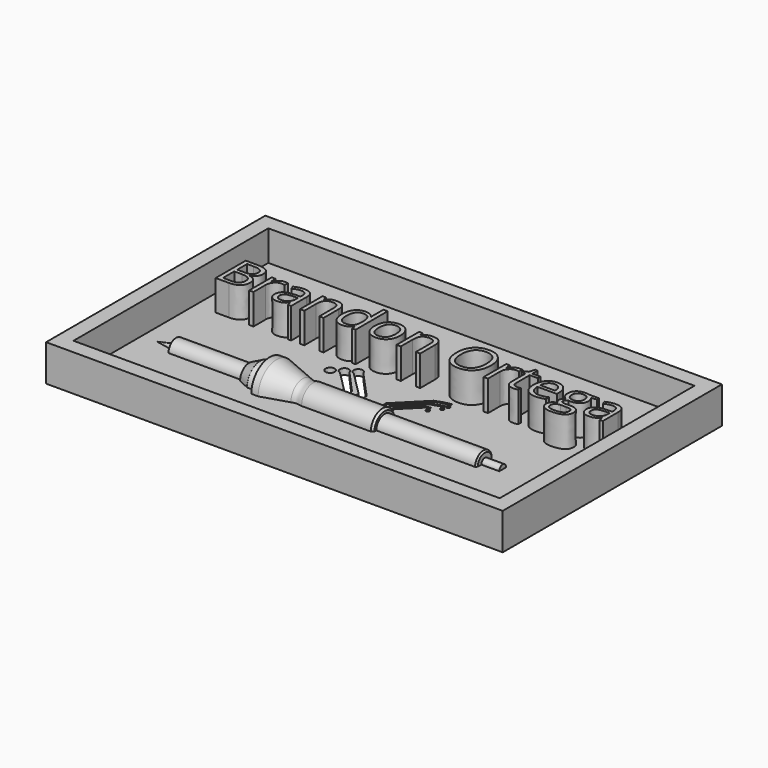
from build123d import *

# Parameters (mm, degrees)
F1_ANGLE     = 180
F0_W         = 2.8489414334
F0_H         = 1.7904182896
F2_ANGLE     = 180
F0_W_2       = 190.5
F0_H_2       = 114.3
F0_W_3       = 177.8
F0_H_3       = 101.6
F0_TEXT_SIZE = 21.9972936401
F3_DEPTH     = 2.54
F4_DEPTH     = 12.7
F5_DEPTH     = 12.7


# Not quite as in the source:
# - Text() gives the source's letters only with a copy of the font that has no kerning and outlines rounded to 1/6400 em; it was checked with that copy


with BuildPart() as f1:
    # F0 (on Top) → F1 (revolve)
    with BuildSketch(Plane.XY):
        with BuildLine():
            Line((-74.5651721954, -13.5963652283), (-82.55, -15.2098201215))
            Line((-82.55, -15.2098201215), (58.8370602846, -15.2098201215))
            Line((58.8370602846, -15.2098201215), (58.8370602846, -13.4194018319))
            Line((58.8370602846, -13.4194018319), (54.2072419855, -13.4194018319))
            Line((54.2072419855, -13.4194018319), (54.2072419855, -11.5678850561))
            Line((54.2072419855, -11.5678850561), (53.6286447975, -10.887705721))
            Line((53.6286447975, -10.887705721), (12.4287380683, -10.887705721))
            Line((12.4287380683, -10.887705721), (12.4287380683, -9.9038422616))
            Line((12.4287380683, -9.9038422616), (11.5140470523, -9.1452874751))
            Line((11.5140470523, -9.1452874751), (7.7323295531, -9.1452874751))
            Line((7.7323295531, -9.1452874751), (6.9703295531, -9.1452874751))
            Line((6.9703295531, -9.1452874751), (5.7003295531, -9.1452874751))
            Line((5.7003295531, -9.1452874751), (4.9383295531, -9.1452874751))
            Line((4.9383295531, -9.1452874751), (3.6683295531, -9.1452874751))
            Line((3.6683295531, -9.1452874751), (2.9063295531, -9.1452874751))
            Line((2.9063295531, -9.1452874751), (-5.1990439205, -9.1452874751))
            Line((-5.1990439205, -9.1452874751), (-8.3740439205, -9.1452874751))
            Line((-8.3740439205, -9.1452874751), (-10.9140439205, -9.1452874751))
            Line((-10.9140439205, -9.1452874751), (-14.0890439205, -9.1452874751))
            Line((-14.0890439205, -9.1452874751), (-16.6290439205, -9.1452874751))
            Line((-16.6290439205, -9.1452874751), (-17.3627614197, -9.1452874751))
            add(Edge.make_bspline(
                [(-21.7048861086, -9.0066427365), (-21.0124520956, -9.19988297), (-19.5884720556, -9.7925185893), (-18.2162617645, -9.1413361473), (-17.3627614197, -9.1452874751)],
                knots=[0, 0, 0, 0, 0.4911919612, 1, 1, 1, 1], degree=3))
            Line((-21.7048861086, -9.0066427365), (-32.662589103, -5.6135384366))
            Line((-32.662589103, -5.6135384366), (-35.5079583824, -5.6135384366))
            Line((-35.5079583824, -5.6135384366), (-35.5079583824, -8.2424543798))
            Line((-35.5079583824, -8.2424543798), (-39.3697954714, -8.2424543798))
            Line((-39.3697954714, -8.2424543798), (-44.1093221307, -10.5244489387))
            Line((-44.1093221307, -10.5244489387), (-44.1093221307, -11.2266018987))
            Line((-44.1093221307, -11.2266018987), (-74.5651721954, -11.2266018987))
            Line((-74.5651721954, -11.2266018987), (-74.5651721954, -13.5963652283))
        make_face()
    revolve(axis=Axis((-11.8564698577, -15.2098201215, 0), (1, 0, 0)), revolution_arc=F1_ANGLE)

    # F0 (on Top) → F2 (revolve)
    with BuildSketch(Plane.XY):
        with Locations((60.2615310013, -14.3146109767)):
            Rectangle(F0_W, F0_H)
    revolve(axis=Axis((60.2615310013, -15.2098201215, 0), (1, 0, 0)), revolution_arc=F2_ANGLE)

    # F0 (on Top) → F3 (join)
    with BuildSketch(Plane.XY):
        Rectangle(F0_W_2, F0_H_2)
        Rectangle(F0_W_3, F0_H_3, mode=Mode.SUBTRACT)
        Rectangle(F0_W_3, F0_H_3)
        with BuildLine():
            Line((-74.5651721954, -16.8232750148), (-82.55, -15.2098201215))
            Line((-82.55, -15.2098201215), (-74.5651721954, -13.5963652283))
            Line((-74.5651721954, -13.5963652283), (-74.5651721954, -11.2266018987))
            Line((-74.5651721954, -11.2266018987), (-44.1093221307, -11.2266018987))
            Line((-44.1093221307, -11.2266018987), (-44.1093221307, -10.5244489387))
            Line((-44.1093221307, -10.5244489387), (-39.3697954714, -8.2424543798))
            Line((-39.3697954714, -8.2424543798), (-35.5079583824, -8.2424543798))
            Line((-35.5079583824, -8.2424543798), (-35.5079583824, -5.6135384366))
            Line((-35.5079583824, -5.6135384366), (-32.662589103, -5.6135384366))
            Line((-32.662589103, -5.6135384366), (-21.7048861086, -9.0066427365))
            add(Edge.make_bspline(
                [(-21.7048861086, -9.0066427365), (-21.0124520956, -9.19988297), (-19.5884720556, -9.7925185893), (-18.2162617645, -9.1413361473), (-17.3627614197, -9.1452874751)],
                knots=[0, 0, 0, 0, 0.4911919612, 1, 1, 1, 1], degree=3))
            Line((-17.3627614197, -9.1452874751), (-16.6290439205, -9.1452874751))
            Line((-16.6290439205, -9.1452874751), (-14.0890439205, -9.1452874751))
            Line((-14.0890439205, -9.1452874751), (-14.0890439205, -3.3032874751))
            Line((-14.0890439205, -3.3032874751), (-22.3246965397, 4.9323651441))
            ThreePointArc((-22.3246965397, 4.9323651441), (-23.2578395891, 8.1815702533), (-20.062313494, 7.0785277481))
            Line((-20.062313494, 7.0785277481), (-10.9140439205, -3.0492874751))
            Line((-10.9140439205, -3.0492874751), (-10.9140439205, -9.1452874751))
            Line((-10.9140439205, -9.1452874751), (-8.3740439205, -9.1452874751))
            Line((-8.3740439205, -9.1452874751), (-8.3740439205, -2.7952874751))
            Line((-8.3740439205, -2.7952874751), (-18.4026051549, 7.2332737592))
            ThreePointArc((-18.4026051549, 7.2332737592), (-19.3413648826, 10.4771416844), (-16.1425614334, 9.3947344434))
            Line((-16.1425614334, 9.3947344434), (-5.1990439205, -2.5412874751))
            Line((-5.1990439205, -2.5412874751), (-5.1990439205, -9.1452874751))
            Line((-5.1990439205, -9.1452874751), (2.9063295531, -9.1452874751))
            Line((2.9063295531, -9.1452874751), (2.9063295531, -2.5412874751))
            Line((2.9063295531, -2.5412874751), (13.9043204597, 8.5183257555))
            Line((13.9043204597, 8.5183257555), (17.1510335058, 9.6937734634))
            Line((17.1510335058, 9.6937734634), (20.0589859507, 10.3021474712))
            Line((20.0589859507, 10.3021474712), (20.2566589924, 9.566233503))
            Line((20.2566589924, 9.566233503), (20.549468061, 8.7620187263))
            ThreePointArc((20.549468061, 8.7620187263), (21.0009293474, 8.5014168437), (21.1792302885, 8.0115807398))
            ThreePointArc((21.1792302885, 8.0115807398), (20.1560011796, 7.2957571913), (19.8343395992, 8.5023785029))
            Line((19.8343395992, 8.5023785029), (19.5207450243, 9.3685604613))
            Line((19.5207450243, 9.3685604613), (17.4104327689, 8.9772847877))
            Line((17.4104327689, 8.9772847877), (14.4446368983, 7.9810198702))
            Line((14.4446368983, 7.9810198702), (3.6683295531, -2.7952874751))
            Line((3.6683295531, -2.7952874751), (3.6683295531, -9.1452874751))
            Line((3.6683295531, -9.1452874751), (4.9383295531, -9.1452874751))
            Line((4.9383295531, -9.1452874751), (4.9383295531, -3.0492874751))
            Line((4.9383295531, -3.0492874751), (14.1417703069, 6.2157840132))
            Line((14.1417703069, 6.2157840132), (17.3898523031, 7.3917273391))
            Line((17.3898523031, 7.3917273391), (19.34044637, 7.947929778))
            Line((19.34044637, 7.947929778), (19.5381194117, 7.2120158098))
            Line((19.5381194117, 7.2120158098), (19.8309284803, 6.4078010331))
            ThreePointArc((19.8309284803, 6.4078010331), (20.2823897667, 6.1471991505), (20.4606907078, 5.6573630466))
            ThreePointArc((20.4606907078, 5.6573630466), (19.4374615989, 4.9415394981), (19.1158000185, 6.1481608097))
            Line((19.1158000185, 6.1481608097), (18.8022054435, 7.014342768))
            Line((18.8022054435, 7.014342768), (17.632497658, 6.6693927685))
            Line((17.632497658, 6.6693927685), (14.6805856741, 5.6769686459))
            Line((14.6805856741, 5.6769686459), (5.7003295531, -3.3032874751))
            Line((5.7003295531, -3.3032874751), (5.7003295531, -9.1452874751))
            Line((5.7003295531, -9.1452874751), (6.9703295531, -9.1452874751))
            Line((6.9703295531, -9.1452874751), (6.9703295531, -3.8112874751))
            Line((6.9703295531, -3.8112874751), (14.3754961374, 3.6554913484))
            Line((14.3754961374, 3.6554913484), (16.3270021512, 4.1796832328))
            Line((16.3270021512, 4.1796832328), (16.524675193, 3.4437692646))
            Line((16.524675193, 3.4437692646), (16.8174842615, 2.6395544879))
            ThreePointArc((16.8174842615, 2.6395544879), (17.2689455479, 2.3789526053), (17.447246489, 1.8891165014))
            ThreePointArc((17.447246489, 1.8891165014), (16.4240173801, 1.1732929529), (16.1023557997, 2.3799142645))
            Line((16.1023557997, 2.3799142645), (15.7887612248, 3.2460962229))
            Line((15.7887612248, 3.2460962229), (14.9165344499, 3.1189174217))
            Line((14.9165344499, 3.1189174217), (7.7323295531, -4.0652874751))
            Line((7.7323295531, -4.0652874751), (7.7323295531, -9.1452874751))
            Line((7.7323295531, -9.1452874751), (11.5140470523, -9.1452874751))
            Line((11.5140470523, -9.1452874751), (12.4287380683, -9.9038422616))
            Line((12.4287380683, -9.9038422616), (12.4287380683, -10.887705721))
            Line((12.4287380683, -10.887705721), (53.6286447975, -10.887705721))
            Line((53.6286447975, -10.887705721), (54.2072419855, -11.5678850561))
            Line((54.2072419855, -11.5678850561), (54.2072419855, -13.4194018319))
            Line((54.2072419855, -13.4194018319), (58.8370602846, -13.4194018319))
            Line((58.8370602846, -13.4194018319), (61.686001718, -13.4194018319))
            Line((61.686001718, -13.4194018319), (61.686001718, -15.2098201215))
            Line((61.686001718, -15.2098201215), (61.686001718, -17.0002384111))
            Line((61.686001718, -17.0002384111), (58.8370602846, -17.0002384111))
            Line((58.8370602846, -17.0002384111), (54.2072419855, -17.0002384111))
            Line((54.2072419855, -17.0002384111), (54.2072419855, -18.8517551869))
            Line((54.2072419855, -18.8517551869), (53.6286447975, -19.5319345221))
            Line((53.6286447975, -19.5319345221), (12.4287380683, -19.5319345221))
            Line((12.4287380683, -19.5319345221), (12.4287380683, -20.5157979815))
            Line((12.4287380683, -20.5157979815), (11.5140470523, -21.2743527679))
            Line((11.5140470523, -21.2743527679), (3.657140649, -21.2743527679))
            Line((3.657140649, -21.2743527679), (2.895140649, -21.2743527679))
            Line((2.895140649, -21.2743527679), (1.625140649, -21.2743527679))
            Line((1.625140649, -21.2743527679), (0.863140649, -21.2743527679))
            Line((0.863140649, -21.2743527679), (-0.406859351, -21.2743527679))
            Line((-0.406859351, -21.2743527679), (-1.168859351, -21.2743527679))
            Line((-1.168859351, -21.2743527679), (-17.3627614197, -21.2743527679))
            add(Edge.make_bspline(
                [(-21.7048861086, -21.4129975066), (-21.0124520956, -21.219757273), (-19.5884720556, -20.6271216538), (-18.2162617645, -21.2783040958), (-17.3627614197, -21.2743527679)],
                knots=[0, 0, 0, 0, 0.4911919612, 1, 1, 1, 1], degree=3))
            Line((-21.7048861086, -21.4129975066), (-32.662589103, -24.8061018065))
            Line((-32.662589103, -24.8061018065), (-35.5079583824, -24.8061018065))
            Line((-35.5079583824, -24.8061018065), (-35.5079583824, -22.1771858633))
            Line((-35.5079583824, -22.1771858633), (-39.3697954714, -22.1771858633))
            Line((-39.3697954714, -22.1771858633), (-44.1093221307, -19.8951913044))
            Line((-44.1093221307, -19.8951913044), (-44.1093221307, -19.1930383444))
            Line((-44.1093221307, -19.1930383444), (-62.366220009, -19.1930383444))
            Line((-62.366220009, -19.1930383444), (-63.128220009, -19.1930383444))
            Line((-63.128220009, -19.1930383444), (-64.398220009, -19.1930383444))
            Line((-64.398220009, -19.1930383444), (-65.160220009, -19.1930383444))
            Line((-65.160220009, -19.1930383444), (-66.430220009, -19.1930383444))
            Line((-66.430220009, -19.1930383444), (-67.192220009, -19.1930383444))
            Line((-67.192220009, -19.1930383444), (-74.5651721954, -19.1930383444))
            Line((-74.5651721954, -19.1930383444), (-74.5651721954, -16.8232750148))
        make_face(mode=Mode.SUBTRACT)
        with BuildLine():
            Line((-80.3915155616, 12.7), (-80.3915155616, 28.4040054127))
            Line((-80.3915155616, 28.4040054127), (-75.9542489851, 28.4040054127))
            add(Edge.make_bspline(
                [(-75.9542489851, 28.4040054127), (-72.8299458728, 28.4040054127), (-71.4327740189, 27.469120433)],
                knots=[0, 0, 0, 1, 1, 1], degree=2))
            add(Edge.make_bspline(
                [(-71.4327740189, 27.469120433), (-70.0356021651, 26.5342354533), (-70.0356021651, 24.5166711773)],
                knots=[0, 0, 0, 1, 1, 1], degree=2))
            add(Edge.make_bspline(
                [(-70.0356021651, 24.5166711773), (-70.0356021651, 23.1177807848), (-70.8141001353, 22.2103924222)],
                knots=[0, 0, 0, 1, 1, 1], degree=2))
            add(Edge.make_bspline(
                [(-70.8141001353, 22.2103924222), (-71.5925981055, 21.3030040595), (-73.0877266576, 21.0349120433)],
                knots=[0, 0, 0, 1, 1, 1], degree=2))
            Line((-73.0877266576, 21.0349120433), (-73.0877266576, 20.9283626522))
            add(Edge.make_bspline(
                [(-73.0877266576, 20.9283626522), (-69.509729364, 20.3165629229), (-69.509729364, 17.1682002706)],
                knots=[0, 0, 0, 1, 1, 1], degree=2))
            add(Edge.make_bspline(
                [(-69.509729364, 17.1682002706), (-69.509729364, 15.0647090663), (-70.9326792963, 13.8823545332)],
                knots=[0, 0, 0, 1, 1, 1], degree=2))
            add(Edge.make_bspline(
                [(-70.9326792963, 13.8823545332), (-72.3556292287, 12.7), (-74.9128146143, 12.7)],
                knots=[0, 0, 0, 1, 1, 1], degree=2))
            Line((-74.9128146143, 12.7), (-80.3915155616, 12.7))
        make_face(mode=Mode.SUBTRACT)
        with BuildLine():
            add(Edge.make_bspline(
                [(-63.0652097429, 24.0646955345), (-62.1406359946, 24.6885250338), (-61.0338971583, 24.6885250338)],
                knots=[0, 0, 0, 1, 1, 1], degree=2))
            add(Edge.make_bspline(
                [(-61.0338971583, 24.6885250338), (-60.2502435724, 24.6885250338), (-59.6281326116, 24.5579161028)],
                knots=[0, 0, 0, 1, 1, 1], degree=2))
            Line((-59.6281326116, 24.5579161028), (-59.8756021651, 22.9046820027))
            add(Edge.make_bspline(
                [(-59.8756021651, 22.9046820027), (-60.6042625169, 23.0662246279), (-61.1645060893, 23.0662246279)],
                knots=[0, 0, 0, 1, 1, 1], degree=2))
            add(Edge.make_bspline(
                [(-61.1645060893, 23.0662246279), (-62.5943301759, 23.0662246279), (-63.6082679296, 21.9062110961)],
                knots=[0, 0, 0, 1, 1, 1], degree=2))
            add(Edge.make_bspline(
                [(-63.6082679296, 21.9062110961), (-64.6222056834, 20.7461975643), (-64.6222056834, 19.0173477673)],
                knots=[0, 0, 0, 1, 1, 1], degree=2))
            Line((-64.6222056834, 19.0173477673), (-64.6222056834, 12.7))
            Line((-64.6222056834, 12.7), (-66.4060487145, 12.7))
            Line((-66.4060487145, 12.7), (-66.4060487145, 24.4719891746))
            Line((-66.4060487145, 24.4719891746), (-64.9349797023, 24.4719891746))
            Line((-64.9349797023, 24.4719891746), (-64.7287550744, 22.2928822733))
            Line((-64.7287550744, 22.2928822733), (-64.6428281461, 22.2928822733))
            add(Edge.make_bspline(
                [(-64.6428281461, 22.2928822733), (-63.9897834912, 23.4408660352), (-63.0652097429, 24.0646955345)],
                knots=[0, 0, 0, 1, 1, 1], degree=2))
        make_face(mode=Mode.SUBTRACT)
        with BuildLine():
            Line((-48.8632070365, 12.7), (-50.1864817321, 12.7))
            Line((-50.1864817321, 12.7), (-50.5405006766, 14.3772936401))
            Line((-50.5405006766, 14.3772936401), (-50.6264276049, 14.3772936401))
            add(Edge.make_bspline(
                [(-50.6264276049, 14.3772936401), (-51.5063193505, 13.2705548038), (-52.3810554804, 12.8770094723)],
                knots=[0, 0, 0, 1, 1, 1], degree=2))
            add(Edge.make_bspline(
                [(-52.3810554804, 12.8770094723), (-53.2557916103, 12.4834641407), (-54.5687550744, 12.4834641407)],
                knots=[0, 0, 0, 1, 1, 1], degree=2))
            add(Edge.make_bspline(
                [(-54.5687550744, 12.4834641407), (-56.3182273342, 12.4834641407), (-57.3115426252, 13.3874154263)],
                knots=[0, 0, 0, 1, 1, 1], degree=2))
            add(Edge.make_bspline(
                [(-57.3115426252, 13.3874154263), (-58.3048579161, 14.2913667118), (-58.3048579161, 15.9549120433)],
                knots=[0, 0, 0, 1, 1, 1], degree=2))
            add(Edge.make_bspline(
                [(-58.3048579161, 15.9549120433), (-58.3048579161, 19.5191610284), (-52.6027469553, 19.691014885)],
                knots=[0, 0, 0, 1, 1, 1], degree=2))
            Line((-52.6027469553, 19.691014885), (-50.6058051421, 19.7563193505))
            Line((-50.6058051421, 19.7563193505), (-50.6058051421, 20.4884167794))
            add(Edge.make_bspline(
                [(-50.6058051421, 20.4884167794), (-50.6058051421, 21.8735588633), (-51.2004194858, 22.5334776725)],
                knots=[0, 0, 0, 1, 1, 1], degree=2))
            add(Edge.make_bspline(
                [(-51.2004194858, 22.5334776725), (-51.7950338295, 23.1933964817), (-53.1079972936, 23.1933964817)],
                knots=[0, 0, 0, 1, 1, 1], degree=2))
            add(Edge.make_bspline(
                [(-53.1079972936, 23.1933964817), (-54.5790663058, 23.1933964817), (-56.4350879567, 22.2928822733)],
                knots=[0, 0, 0, 1, 1, 1], degree=2))
            Line((-56.4350879567, 22.2928822733), (-56.9850202977, 23.6574018945))
            add(Edge.make_bspline(
                [(-56.9850202977, 23.6574018945), (-56.1154397835, 24.1282814614), (-55.0791610284, 24.3963734777)],
                knots=[0, 0, 0, 1, 1, 1], degree=2))
            add(Edge.make_bspline(
                [(-55.0791610284, 24.3963734777), (-54.0428822733, 24.6644654939), (-52.9980108254, 24.6644654939)],
                knots=[0, 0, 0, 1, 1, 1], degree=2))
            add(Edge.make_bspline(
                [(-52.9980108254, 24.6644654939), (-50.8945196211, 24.6644654939), (-49.8788633288, 23.7312990528)],
                knots=[0, 0, 0, 1, 1, 1], degree=2))
            add(Edge.make_bspline(
                [(-49.8788633288, 23.7312990528), (-48.8632070365, 22.7981326116), (-48.8632070365, 20.7358863329)],
                knots=[0, 0, 0, 1, 1, 1], degree=2))
            Line((-48.8632070365, 20.7358863329), (-48.8632070365, 12.7))
        make_face(mode=Mode.SUBTRACT)
        with BuildLine():
            ThreePointArc((-26.2389803515, 2.3696489559), (-27.1644583182, 5.626112764), (-23.9736375963, 4.4948616332))
            ThreePointArc((-23.9736375963, 4.4948616332), (-23.960471465, 4.3661239156), (-23.9560759934, 4.236789362))
            ThreePointArc((-23.9560759934, 4.236789362), (-24.6550251657, 2.7621821597), (-26.2389803515, 2.3696489559))
        make_face(mode=Mode.SUBTRACT)
        with BuildLine():
            Line((-35.3520568336, 12.7), (-37.1358998647, 12.7))
            Line((-37.1358998647, 12.7), (-37.1358998647, 20.3165629229))
            add(Edge.make_bspline(
                [(-37.1358998647, 20.3165629229), (-37.1358998647, 21.7532611637), (-37.7906630582, 22.4630175913)],
                knots=[0, 0, 0, 1, 1, 1], degree=2))
            add(Edge.make_bspline(
                [(-37.7906630582, 22.4630175913), (-38.4454262517, 23.1727740189), (-39.8443166441, 23.1727740189)],
                knots=[0, 0, 0, 1, 1, 1], degree=2))
            add(Edge.make_bspline(
                [(-39.8443166441, 23.1727740189), (-41.6900270636, 23.1727740189), (-42.5492963464, 22.1743031123)],
                knots=[0, 0, 0, 1, 1, 1], degree=2))
            add(Edge.make_bspline(
                [(-42.5492963464, 22.1743031123), (-43.4085656292, 21.1758322057), (-43.4085656292, 18.8764276049)],
                knots=[0, 0, 0, 1, 1, 1], degree=2))
            Line((-43.4085656292, 18.8764276049), (-43.4085656292, 12.7))
            Line((-43.4085656292, 12.7), (-45.1924086604, 12.7))
            Line((-45.1924086604, 12.7), (-45.1924086604, 24.4719891746))
            Line((-45.1924086604, 24.4719891746), (-43.741962111, 24.4719891746))
            Line((-43.741962111, 24.4719891746), (-43.4532476319, 22.86))
            Line((-43.4532476319, 22.86), (-43.3673207037, 22.86))
            add(Edge.make_bspline(
                [(-43.3673207037, 22.86), (-42.8173883627, 23.7295805142), (-41.8292286874, 24.209052774)],
                knots=[0, 0, 0, 1, 1, 1], degree=2))
            add(Edge.make_bspline(
                [(-41.8292286874, 24.209052774), (-40.8410690122, 24.6885250338), (-39.6277807848, 24.6885250338)],
                knots=[0, 0, 0, 1, 1, 1], degree=2))
            add(Edge.make_bspline(
                [(-39.6277807848, 24.6885250338), (-37.5002300406, 24.6885250338), (-36.4261434371, 23.6625575101)],
                knots=[0, 0, 0, 1, 1, 1], degree=2))
            add(Edge.make_bspline(
                [(-36.4261434371, 23.6625575101), (-35.3520568336, 22.6365899865), (-35.3520568336, 20.3784303112)],
                knots=[0, 0, 0, 1, 1, 1], degree=2))
            Line((-35.3520568336, 20.3784303112), (-35.3520568336, 12.7))
        make_face(mode=Mode.SUBTRACT)
        with BuildLine():
            Line((-23.4425845737, 12.7), (-23.6797428958, 14.2776184032))
            Line((-23.6797428958, 14.2776184032), (-23.7759810555, 14.2776184032))
            add(Edge.make_bspline(
                [(-23.7759810555, 14.2776184032), (-25.0098917456, 12.4834641407), (-27.4708389716, 12.4834641407)],
                knots=[0, 0, 0, 1, 1, 1], degree=2))
            add(Edge.make_bspline(
                [(-27.4708389716, 12.4834641407), (-29.7805548038, 12.4834641407), (-31.0643031123, 14.0628010825)],
                knots=[0, 0, 0, 1, 1, 1], degree=2))
            add(Edge.make_bspline(
                [(-31.0643031123, 14.0628010825), (-32.3480514208, 15.6421380244), (-32.3480514208, 18.5533423545)],
                knots=[0, 0, 0, 1, 1, 1], degree=2))
            add(Edge.make_bspline(
                [(-32.3480514208, 18.5533423545), (-32.3480514208, 21.4645466847), (-31.0591474966, 23.0765358593)],
                knots=[0, 0, 0, 1, 1, 1], degree=2))
            add(Edge.make_bspline(
                [(-31.0591474966, 23.0765358593), (-29.7702435724, 24.6885250338), (-27.4708389716, 24.6885250338)],
                knots=[0, 0, 0, 1, 1, 1], degree=2))
            add(Edge.make_bspline(
                [(-27.4708389716, 24.6885250338), (-25.0751962111, 24.6885250338), (-23.7966035183, 22.9459269283)],
                knots=[0, 0, 0, 1, 1, 1], degree=2))
            Line((-23.7966035183, 22.9459269283), (-23.6556833559, 22.9459269283))
            Line((-23.6556833559, 22.9459269283), (-23.7312990528, 23.7948849797))
            Line((-23.7312990528, 23.7948849797), (-23.7759810555, 24.6232205683))
            Line((-23.7759810555, 24.6232205683), (-23.7759810555, 29.4145060893))
            Line((-23.7759810555, 29.4145060893), (-21.9921380244, 29.4145060893))
            Line((-21.9921380244, 29.4145060893), (-21.9921380244, 12.7))
            Line((-21.9921380244, 12.7), (-23.4425845737, 12.7))
        make_face(mode=Mode.SUBTRACT)
        with BuildLine():
            add(Edge.make_bspline(
                [(-9.5069553451, 23.0438836265), (-8.05135318, 21.3992422192), (-8.05135318, 18.5980243572)],
                knots=[0, 0, 0, 1, 1, 1], degree=2))
            add(Edge.make_bspline(
                [(-8.05135318, 18.5980243572), (-8.05135318, 15.7177537212), (-9.5000811908, 14.100608931)],
                knots=[0, 0, 0, 1, 1, 1], degree=2))
            add(Edge.make_bspline(
                [(-9.5000811908, 14.100608931), (-10.9488092016, 12.4834641407), (-13.5059945873, 12.4834641407)],
                knots=[0, 0, 0, 1, 1, 1], degree=2))
            add(Edge.make_bspline(
                [(-13.5059945873, 12.4834641407), (-15.0870500677, 12.4834641407), (-16.3106495264, 13.2258728011)],
                knots=[0, 0, 0, 1, 1, 1], degree=2))
            add(Edge.make_bspline(
                [(-16.3106495264, 13.2258728011), (-17.5342489851, 13.9682814614), (-18.2010419486, 15.3534235453)],
                knots=[0, 0, 0, 1, 1, 1], degree=2))
            add(Edge.make_bspline(
                [(-18.2010419486, 15.3534235453), (-18.867834912, 16.7385656292), (-18.867834912, 18.5980243572)],
                knots=[0, 0, 0, 1, 1, 1], degree=2))
            add(Edge.make_bspline(
                [(-18.867834912, 18.5980243572), (-18.867834912, 21.4748579161), (-17.427699594, 23.081691475)],
                knots=[0, 0, 0, 1, 1, 1], degree=2))
            add(Edge.make_bspline(
                [(-17.427699594, 23.081691475), (-15.987564276, 24.6885250338), (-13.4303788904, 24.6885250338)],
                knots=[0, 0, 0, 1, 1, 1], degree=2))
            add(Edge.make_bspline(
                [(-13.4303788904, 24.6885250338), (-10.9625575101, 24.6885250338), (-9.5069553451, 23.0438836265)],
                knots=[0, 0, 0, 1, 1, 1], degree=2))
        make_face(mode=Mode.SUBTRACT)
        with BuildLine():
            Line((4.9167388363, 12.7), (3.1328958051, 12.7))
            Line((3.1328958051, 12.7), (3.1328958051, 20.3165629229))
            add(Edge.make_bspline(
                [(3.1328958051, 20.3165629229), (3.1328958051, 21.7532611637), (2.4781326116, 22.4630175913)],
                knots=[0, 0, 0, 1, 1, 1], degree=2))
            add(Edge.make_bspline(
                [(2.4781326116, 22.4630175913), (1.8233694181, 23.1727740189), (0.4244790257, 23.1727740189)],
                knots=[0, 0, 0, 1, 1, 1], degree=2))
            add(Edge.make_bspline(
                [(0.4244790257, 23.1727740189), (-1.4212313938, 23.1727740189), (-2.2805006766, 22.1743031123)],
                knots=[0, 0, 0, 1, 1, 1], degree=2))
            add(Edge.make_bspline(
                [(-2.2805006766, 22.1743031123), (-3.1397699594, 21.1758322057), (-3.1397699594, 18.8764276049)],
                knots=[0, 0, 0, 1, 1, 1], degree=2))
            Line((-3.1397699594, 18.8764276049), (-3.1397699594, 12.7))
            Line((-3.1397699594, 12.7), (-4.9236129905, 12.7))
            Line((-4.9236129905, 12.7), (-4.9236129905, 24.4719891746))
            Line((-4.9236129905, 24.4719891746), (-3.4731664411, 24.4719891746))
            Line((-3.4731664411, 24.4719891746), (-3.1844519621, 22.86))
            Line((-3.1844519621, 22.86), (-3.0985250338, 22.86))
            add(Edge.make_bspline(
                [(-3.0985250338, 22.86), (-2.5485926928, 23.7295805142), (-1.5604330176, 24.209052774)],
                knots=[0, 0, 0, 1, 1, 1], degree=2))
            add(Edge.make_bspline(
                [(-1.5604330176, 24.209052774), (-0.5722733424, 24.6885250338), (0.641014885, 24.6885250338)],
                knots=[0, 0, 0, 1, 1, 1], degree=2))
            add(Edge.make_bspline(
                [(0.641014885, 24.6885250338), (2.7685656292, 24.6885250338), (3.8426522327, 23.6625575101)],
                knots=[0, 0, 0, 1, 1, 1], degree=2))
            add(Edge.make_bspline(
                [(3.8426522327, 23.6625575101), (4.9167388363, 22.6365899865), (4.9167388363, 20.3784303112)],
                knots=[0, 0, 0, 1, 1, 1], degree=2))
            Line((4.9167388363, 20.3784303112), (4.9167388363, 12.7))
        make_face(mode=Mode.SUBTRACT)
        with BuildLine():
            add(Edge.make_bspline(
                [(26.2919215156, 26.5033017591), (28.1926251691, 24.3551285521), (28.1926251691, 20.5743437077)],
                knots=[0, 0, 0, 1, 1, 1], degree=2))
            add(Edge.make_bspline(
                [(28.1926251691, 20.5743437077), (28.1926251691, 16.8038700947), (26.2850473613, 14.6436671177)],
                knots=[0, 0, 0, 1, 1, 1], degree=2))
            add(Edge.make_bspline(
                [(26.2850473613, 14.6436671177), (24.3774695535, 12.4834641407), (20.9850744249, 12.4834641407)],
                knots=[0, 0, 0, 1, 1, 1], degree=2))
            add(Edge.make_bspline(
                [(20.9850744249, 12.4834641407), (17.5170635995, 12.4834641407), (15.631826793, 14.6058592693)],
                knots=[0, 0, 0, 1, 1, 1], degree=2))
            add(Edge.make_bspline(
                [(15.631826793, 14.6058592693), (13.7465899865, 16.7282543978), (13.7465899865, 20.5949661705)],
                knots=[0, 0, 0, 1, 1, 1], degree=2))
            add(Edge.make_bspline(
                [(13.7465899865, 20.5949661705), (13.7465899865, 24.430744249), (15.6369824087, 26.5411096076)],
                knots=[0, 0, 0, 1, 1, 1], degree=2))
            add(Edge.make_bspline(
                [(15.6369824087, 26.5411096076), (17.5273748309, 28.6514749662), (21.0056968877, 28.6514749662)],
                knots=[0, 0, 0, 1, 1, 1], degree=2))
            add(Edge.make_bspline(
                [(21.0056968877, 28.6514749662), (24.391217862, 28.6514749662), (26.2919215156, 26.5033017591)],
                knots=[0, 0, 0, 1, 1, 1], degree=2))
        make_face(mode=Mode.SUBTRACT)
        with BuildLine():
            add(Edge.make_bspline(
                [(34.7643166441, 24.0646955345), (35.6888903924, 24.6885250338), (36.7956292287, 24.6885250338)],
                knots=[0, 0, 0, 1, 1, 1], degree=2))
            add(Edge.make_bspline(
                [(36.7956292287, 24.6885250338), (37.5792828146, 24.6885250338), (38.2013937754, 24.5579161028)],
                knots=[0, 0, 0, 1, 1, 1], degree=2))
            Line((38.2013937754, 24.5579161028), (37.9539242219, 22.9046820027))
            add(Edge.make_bspline(
                [(37.9539242219, 22.9046820027), (37.2252638701, 23.0662246279), (36.6650202977, 23.0662246279)],
                knots=[0, 0, 0, 1, 1, 1], degree=2))
            add(Edge.make_bspline(
                [(36.6650202977, 23.0662246279), (35.2351962111, 23.0662246279), (34.2212584574, 21.9062110961)],
                knots=[0, 0, 0, 1, 1, 1], degree=2))
            add(Edge.make_bspline(
                [(34.2212584574, 21.9062110961), (33.2073207037, 20.7461975643), (33.2073207037, 19.0173477673)],
                knots=[0, 0, 0, 1, 1, 1], degree=2))
            Line((33.2073207037, 19.0173477673), (33.2073207037, 12.7))
            Line((33.2073207037, 12.7), (31.4234776725, 12.7))
            Line((31.4234776725, 12.7), (31.4234776725, 24.4719891746))
            Line((31.4234776725, 24.4719891746), (32.8945466847, 24.4719891746))
            Line((32.8945466847, 24.4719891746), (33.1007713126, 22.2928822733))
            Line((33.1007713126, 22.2928822733), (33.1866982409, 22.2928822733))
            add(Edge.make_bspline(
                [(33.1866982409, 22.2928822733), (33.8397428958, 23.4408660352), (34.7643166441, 24.0646955345)],
                knots=[0, 0, 0, 1, 1, 1], degree=2))
        make_face(mode=Mode.SUBTRACT)
        with BuildLine():
            add(Edge.make_bspline(
                [(42.8208254398, 14.5268064953), (43.3260757781, 13.95797023), (44.2059675237, 13.95797023)],
                knots=[0, 0, 0, 1, 1, 1], degree=2))
            add(Edge.make_bspline(
                [(44.2059675237, 13.95797023), (44.6802841678, 13.95797023), (45.1202300406, 14.0267117727)],
                knots=[0, 0, 0, 1, 1, 1], degree=2))
            add(Edge.make_bspline(
                [(45.1202300406, 14.0267117727), (45.5601759134, 14.0954533153), (45.8179566982, 14.1710690122)],
                knots=[0, 0, 0, 1, 1, 1], degree=2))
            Line((45.8179566982, 14.1710690122), (45.8179566982, 12.8065493911))
            add(Edge.make_bspline(
                [(45.8179566982, 12.8065493911), (45.5292422192, 12.6690663058), (44.9655615697, 12.5762652233)],
                knots=[0, 0, 0, 1, 1, 1], degree=2))
            add(Edge.make_bspline(
                [(44.9655615697, 12.5762652233), (44.4018809202, 12.4834641407), (43.9481867388, 12.4834641407)],
                knots=[0, 0, 0, 1, 1, 1], degree=2))
            add(Edge.make_bspline(
                [(43.9481867388, 12.4834641407), (40.5351691475, 12.4834641407), (40.5351691475, 16.0820838972)],
                knots=[0, 0, 0, 1, 1, 1], degree=2))
            Line((40.5351691475, 16.0820838972), (40.5351691475, 23.0868470907))
            Line((40.5351691475, 23.0868470907), (38.847564276, 23.0868470907))
            Line((38.847564276, 23.0868470907), (38.847564276, 23.9461163735))
            Line((38.847564276, 23.9461163735), (40.5351691475, 24.6885250338))
            Line((40.5351691475, 24.6885250338), (41.2844519621, 27.2010284168))
            Line((41.2844519621, 27.2010284168), (42.3155751015, 27.2010284168))
            Line((42.3155751015, 27.2010284168), (42.3155751015, 24.4719891746))
            Line((42.3155751015, 24.4719891746), (45.73202977, 24.4719891746))
            Line((45.73202977, 24.4719891746), (45.73202977, 23.0868470907))
            Line((45.73202977, 23.0868470907), (42.3155751015, 23.0868470907))
            Line((42.3155751015, 23.0868470907), (42.3155751015, 16.157699594))
            add(Edge.make_bspline(
                [(42.3155751015, 16.157699594), (42.3155751015, 15.0956427605), (42.8208254398, 14.5268064953)],
                knots=[0, 0, 0, 1, 1, 1], degree=2))
        make_face(mode=Mode.SUBTRACT)
        with BuildLine():
            add(Edge.make_bspline(
                [(55.1771177267, 12.6621921516), (54.3350338295, 12.4834641407), (53.142368065, 12.4834641407)],
                knots=[0, 0, 0, 1, 1, 1], degree=2))
            add(Edge.make_bspline(
                [(53.142368065, 12.4834641407), (50.5336265223, 12.4834641407), (49.0230311231, 14.0748308525)],
                knots=[0, 0, 0, 1, 1, 1], degree=2))
            add(Edge.make_bspline(
                [(49.0230311231, 14.0748308525), (47.512435724, 15.6661975643), (47.512435724, 18.488037889)],
                knots=[0, 0, 0, 1, 1, 1], degree=2))
            add(Edge.make_bspline(
                [(47.512435724, 18.488037889), (47.512435724, 21.3373748309), (48.9147631935, 23.0129499323)],
                knots=[0, 0, 0, 1, 1, 1], degree=2))
            add(Edge.make_bspline(
                [(48.9147631935, 23.0129499323), (50.3170906631, 24.6885250338), (52.6817997294, 24.6885250338)],
                knots=[0, 0, 0, 1, 1, 1], degree=2))
            add(Edge.make_bspline(
                [(52.6817997294, 24.6885250338), (54.8918403248, 24.6885250338), (56.180744249, 23.2329228687)],
                knots=[0, 0, 0, 1, 1, 1], degree=2))
            add(Edge.make_bspline(
                [(56.180744249, 23.2329228687), (57.4696481732, 21.7773207037), (57.4696481732, 19.3919891746)],
                knots=[0, 0, 0, 1, 1, 1], degree=2))
            Line((57.4696481732, 19.3919891746), (57.4696481732, 18.2646278755))
            Line((57.4696481732, 18.2646278755), (49.3615832206, 18.2646278755))
            add(Edge.make_bspline(
                [(49.3615832206, 18.2646278755), (49.4165764547, 16.1920703654), (50.4098917456, 15.1179837618)],
                knots=[0, 0, 0, 1, 1, 1], degree=2))
            add(Edge.make_bspline(
                [(50.4098917456, 15.1179837618), (51.4032070365, 14.0438971583), (53.2076725304, 14.0438971583)],
                knots=[0, 0, 0, 1, 1, 1], degree=2))
            add(Edge.make_bspline(
                [(53.2076725304, 14.0438971583), (55.108376184, 14.0438971583), (56.9643978349, 14.8378619756)],
                knots=[0, 0, 0, 1, 1, 1], degree=2))
            Line((56.9643978349, 14.8378619756), (56.9643978349, 13.2464952639))
            add(Edge.make_bspline(
                [(56.9643978349, 13.2464952639), (56.0192016238, 12.8409201624), (55.1771177267, 12.6621921516)],
                knots=[0, 0, 0, 1, 1, 1], degree=2))
        make_face(mode=Mode.SUBTRACT)
        with BuildLine():
            Line((66.0760893099, 24.4719891746), (70.1455886333, 24.4719891746))
            Line((70.1455886333, 24.4719891746), (70.1455886333, 23.3446278755))
            Line((70.1455886333, 23.3446278755), (67.9664817321, 23.0868470907))
            add(Edge.make_bspline(
                [(67.9664817321, 23.0868470907), (68.2655074425, 22.7122056834), (68.5026657645, 22.1038430311)],
                knots=[0, 0, 0, 1, 1, 1], degree=2))
            add(Edge.make_bspline(
                [(68.5026657645, 22.1038430311), (68.7398240866, 21.4954803789), (68.7398240866, 20.7358863329)],
                knots=[0, 0, 0, 1, 1, 1], degree=2))
            add(Edge.make_bspline(
                [(68.7398240866, 20.7358863329), (68.7398240866, 19.0035994587), (67.5574695535, 17.9724763194)],
                knots=[0, 0, 0, 1, 1, 1], degree=2))
            add(Edge.make_bspline(
                [(67.5574695535, 17.9724763194), (66.3751150203, 16.94135318), (64.3128687415, 16.94135318)],
                knots=[0, 0, 0, 1, 1, 1], degree=2))
            add(Edge.make_bspline(
                [(64.3128687415, 16.94135318), (63.7869959405, 16.94135318), (63.3264276049, 17.0272801083)],
                knots=[0, 0, 0, 1, 1, 1], degree=2))
            add(Edge.make_bspline(
                [(63.3264276049, 17.0272801083), (62.1887550744, 16.4257916103), (62.1887550744, 15.5149661705)],
                knots=[0, 0, 0, 1, 1, 1], degree=2))
            add(Edge.make_bspline(
                [(62.1887550744, 15.5149661705), (62.1887550744, 15.030338295), (62.5857374831, 14.8000541272)],
                knots=[0, 0, 0, 1, 1, 1], degree=2))
            add(Edge.make_bspline(
                [(62.5857374831, 14.8000541272), (62.9827198917, 14.5697699594), (63.9485385656, 14.5697699594)],
                knots=[0, 0, 0, 1, 1, 1], degree=2))
            Line((63.9485385656, 14.5697699594), (66.0314073072, 14.5697699594))
            add(Edge.make_bspline(
                [(66.0314073072, 14.5697699594), (67.9458592693, 14.5697699594), (68.9701082544, 13.7637753721)],
                knots=[0, 0, 0, 1, 1, 1], degree=2))
            add(Edge.make_bspline(
                [(68.9701082544, 13.7637753721), (69.9943572395, 12.9577807848), (69.9943572395, 11.4214073072)],
                knots=[0, 0, 0, 1, 1, 1], degree=2))
            add(Edge.make_bspline(
                [(69.9943572395, 11.4214073072), (69.9943572395, 9.4657104195), (68.4270500677, 8.4397428958)],
                knots=[0, 0, 0, 1, 1, 1], degree=2))
            add(Edge.make_bspline(
                [(68.4270500677, 8.4397428958), (66.8597428958, 7.4137753721), (63.852300406, 7.4137753721)],
                knots=[0, 0, 0, 1, 1, 1], degree=2))
            add(Edge.make_bspline(
                [(63.852300406, 7.4137753721), (61.5425845737, 7.4137753721), (60.291488498, 8.2730446549)],
                knots=[0, 0, 0, 1, 1, 1], degree=2))
            add(Edge.make_bspline(
                [(60.291488498, 8.2730446549), (59.0403924222, 9.1323139378), (59.0403924222, 10.7030581867)],
                knots=[0, 0, 0, 1, 1, 1], degree=2))
            add(Edge.make_bspline(
                [(59.0403924222, 10.7030581867), (59.0403924222, 11.7754262517), (59.7278078484, 12.5607983762)],
                knots=[0, 0, 0, 1, 1, 1], degree=2))
            add(Edge.make_bspline(
                [(59.7278078484, 12.5607983762), (60.4152232747, 13.3461705007), (61.6594451962, 13.6245737483)],
                knots=[0, 0, 0, 1, 1, 1], degree=2))
            add(Edge.make_bspline(
                [(61.6594451962, 13.6245737483), (61.209188092, 13.8273612991), (60.9032882273, 14.2569959405)],
                knots=[0, 0, 0, 1, 1, 1], degree=2))
            add(Edge.make_bspline(
                [(60.9032882273, 14.2569959405), (60.5973883627, 14.6866305819), (60.5973883627, 15.2571853857)],
                knots=[0, 0, 0, 1, 1, 1], degree=2))
            add(Edge.make_bspline(
                [(60.5973883627, 15.2571853857), (60.5973883627, 15.8999188092), (60.9410960758, 16.3845466847)],
                knots=[0, 0, 0, 1, 1, 1], degree=2))
            add(Edge.make_bspline(
                [(60.9410960758, 16.3845466847), (61.2848037889, 16.8691745602), (62.0272124493, 17.3194316644)],
                knots=[0, 0, 0, 1, 1, 1], degree=2))
            add(Edge.make_bspline(
                [(62.0272124493, 17.3194316644), (61.1129499323, 17.6940730717), (60.5389580514, 18.5963058187)],
                knots=[0, 0, 0, 1, 1, 1], degree=2))
            add(Edge.make_bspline(
                [(60.5389580514, 18.5963058187), (59.9649661705, 19.4985385656), (59.9649661705, 20.660270636)],
                knots=[0, 0, 0, 1, 1, 1], degree=2))
            add(Edge.make_bspline(
                [(59.9649661705, 20.660270636), (59.9649661705, 22.5919079838), (61.1249797023, 23.6402165088)],
                knots=[0, 0, 0, 1, 1, 1], degree=2))
            add(Edge.make_bspline(
                [(61.1249797023, 23.6402165088), (62.2849932341, 24.6885250338), (64.4091069012, 24.6885250338)],
                knots=[0, 0, 0, 1, 1, 1], degree=2))
            add(Edge.make_bspline(
                [(64.4091069012, 24.6885250338), (65.3336806495, 24.6885250338), (66.0760893099, 24.4719891746)],
                knots=[0, 0, 0, 1, 1, 1], degree=2))
        make_face(mode=Mode.SUBTRACT)
        with BuildLine():
            Line((81.1236129905, 12.7), (79.800338295, 12.7))
            Line((79.800338295, 12.7), (79.4463193505, 14.3772936401))
            Line((79.4463193505, 14.3772936401), (79.3603924222, 14.3772936401))
            add(Edge.make_bspline(
                [(79.3603924222, 14.3772936401), (78.4805006766, 13.2705548038), (77.6057645467, 12.8770094723)],
                knots=[0, 0, 0, 1, 1, 1], degree=2))
            add(Edge.make_bspline(
                [(77.6057645467, 12.8770094723), (76.7310284168, 12.4834641407), (75.4180649526, 12.4834641407)],
                knots=[0, 0, 0, 1, 1, 1], degree=2))
            add(Edge.make_bspline(
                [(75.4180649526, 12.4834641407), (73.6685926928, 12.4834641407), (72.6752774019, 13.3874154263)],
                knots=[0, 0, 0, 1, 1, 1], degree=2))
            add(Edge.make_bspline(
                [(72.6752774019, 13.3874154263), (71.681962111, 14.2913667118), (71.681962111, 15.9549120433)],
                knots=[0, 0, 0, 1, 1, 1], degree=2))
            add(Edge.make_bspline(
                [(71.681962111, 15.9549120433), (71.681962111, 19.5191610284), (77.3840730717, 19.691014885)],
                knots=[0, 0, 0, 1, 1, 1], degree=2))
            Line((77.3840730717, 19.691014885), (79.381014885, 19.7563193505))
            Line((79.381014885, 19.7563193505), (79.381014885, 20.4884167794))
            add(Edge.make_bspline(
                [(79.381014885, 20.4884167794), (79.381014885, 21.8735588633), (78.7864005413, 22.5334776725)],
                knots=[0, 0, 0, 1, 1, 1], degree=2))
            add(Edge.make_bspline(
                [(78.7864005413, 22.5334776725), (78.1917861976, 23.1933964817), (76.8788227334, 23.1933964817)],
                knots=[0, 0, 0, 1, 1, 1], degree=2))
            add(Edge.make_bspline(
                [(76.8788227334, 23.1933964817), (75.4077537212, 23.1933964817), (73.5517320704, 22.2928822733)],
                knots=[0, 0, 0, 1, 1, 1], degree=2))
            Line((73.5517320704, 22.2928822733), (73.0017997294, 23.6574018945))
            add(Edge.make_bspline(
                [(73.0017997294, 23.6574018945), (73.8713802436, 24.1282814614), (74.9076589986, 24.3963734777)],
                knots=[0, 0, 0, 1, 1, 1], degree=2))
            add(Edge.make_bspline(
                [(74.9076589986, 24.3963734777), (75.9439377537, 24.6644654939), (76.9888092016, 24.6644654939)],
                knots=[0, 0, 0, 1, 1, 1], degree=2))
            add(Edge.make_bspline(
                [(76.9888092016, 24.6644654939), (79.092300406, 24.6644654939), (80.1079566982, 23.7312990528)],
                knots=[0, 0, 0, 1, 1, 1], degree=2))
            add(Edge.make_bspline(
                [(80.1079566982, 23.7312990528), (81.1236129905, 22.7981326116), (81.1236129905, 20.7358863329)],
                knots=[0, 0, 0, 1, 1, 1], degree=2))
            Line((81.1236129905, 20.7358863329), (81.1236129905, 12.7))
        make_face(mode=Mode.SUBTRACT)
        with BuildLine():
            add(Edge.make_bspline(
                [(17.0375913396, 25.3690663058), (15.6782273342, 23.7192692828), (15.6782273342, 20.5743437077)],
                knots=[0, 0, 0, 1, 1, 1], degree=2))
            add(Edge.make_bspline(
                [(15.6782273342, 20.5743437077), (15.6782273342, 17.3847361299), (17.0375913396, 15.7349391069)],
                knots=[0, 0, 0, 1, 1, 1], degree=2))
            add(Edge.make_bspline(
                [(17.0375913396, 15.7349391069), (18.3969553451, 14.0851420839), (20.9850744249, 14.0851420839)],
                knots=[0, 0, 0, 1, 1, 1], degree=2))
            add(Edge.make_bspline(
                [(20.9850744249, 14.0851420839), (23.5938159675, 14.0851420839), (24.9256833559, 15.7280649526)],
                knots=[0, 0, 0, 1, 1, 1], degree=2))
            add(Edge.make_bspline(
                [(24.9256833559, 15.7280649526), (26.2575507442, 17.3709878214), (26.2575507442, 20.5743437077)],
                knots=[0, 0, 0, 1, 1, 1], degree=2))
            add(Edge.make_bspline(
                [(26.2575507442, 20.5743437077), (26.2575507442, 23.7433288227), (24.9308389716, 25.3810960758)],
                knots=[0, 0, 0, 1, 1, 1], degree=2))
            add(Edge.make_bspline(
                [(24.9308389716, 25.3810960758), (23.6041271989, 27.0188633288), (21.0056968877, 27.0188633288)],
                knots=[0, 0, 0, 1, 1, 1], degree=2))
            add(Edge.make_bspline(
                [(21.0056968877, 27.0188633288), (18.3969553451, 27.0188633288), (17.0375913396, 25.3690663058)],
                knots=[0, 0, 0, 1, 1, 1], degree=2))
        make_face()
        with BuildLine():
            add(Edge.make_bspline(
                [(-16.1267658999, 22.0230717185), (-17.0186874154, 20.8733694181), (-17.0186874154, 18.5980243572)],
                knots=[0, 0, 0, 1, 1, 1], degree=2))
            add(Edge.make_bspline(
                [(-17.0186874154, 18.5980243572), (-17.0186874154, 16.339864682), (-16.1164546685, 15.1592286874)],
                knots=[0, 0, 0, 1, 1, 1], degree=2))
            add(Edge.make_bspline(
                [(-16.1164546685, 15.1592286874), (-15.2142219215, 13.9785926928), (-13.4647496617, 13.9785926928)],
                knots=[0, 0, 0, 1, 1, 1], degree=2))
            add(Edge.make_bspline(
                [(-13.4647496617, 13.9785926928), (-11.7118403248, 13.9785926928), (-10.8044519621, 15.1540730717)],
                knots=[0, 0, 0, 1, 1, 1], degree=2))
            add(Edge.make_bspline(
                [(-10.8044519621, 15.1540730717), (-9.8970635995, 16.3295534506), (-9.8970635995, 18.5980243572)],
                knots=[0, 0, 0, 1, 1, 1], degree=2))
            add(Edge.make_bspline(
                [(-9.8970635995, 18.5980243572), (-9.8970635995, 20.842435724), (-10.8044519621, 22.0076048714)],
                knots=[0, 0, 0, 1, 1, 1], degree=2))
            add(Edge.make_bspline(
                [(-10.8044519621, 22.0076048714), (-11.7118403248, 23.1727740189), (-13.4853721245, 23.1727740189)],
                knots=[0, 0, 0, 1, 1, 1], degree=2))
            add(Edge.make_bspline(
                [(-13.4853721245, 23.1727740189), (-15.2348443843, 23.1727740189), (-16.1267658999, 22.0230717185)],
                knots=[0, 0, 0, 1, 1, 1], degree=2))
        make_face()
        with BuildLine():
            add(Edge.make_bspline(
                [(-29.6722868742, 15.1282949932), (-28.8456698241, 13.9785926928), (-27.2439918809, 13.9785926928)],
                knots=[0, 0, 0, 1, 1, 1], degree=2))
            add(Edge.make_bspline(
                [(-27.2439918809, 13.9785926928), (-25.4189039242, 13.9785926928), (-24.5974424899, 14.9719079838)],
                knots=[0, 0, 0, 1, 1, 1], degree=2))
            add(Edge.make_bspline(
                [(-24.5974424899, 14.9719079838), (-23.7759810555, 15.9652232747), (-23.7759810555, 18.1787009472)],
                knots=[0, 0, 0, 1, 1, 1], degree=2))
            Line((-23.7759810555, 18.1787009472), (-23.7759810555, 18.5533423545))
            add(Edge.make_bspline(
                [(-23.7759810555, 18.5533423545), (-23.7759810555, 21.0555345061), (-24.6077537212, 22.1244654939)],
                knots=[0, 0, 0, 1, 1, 1], degree=2))
            add(Edge.make_bspline(
                [(-24.6077537212, 22.1244654939), (-25.439526387, 23.1933964817), (-27.2646143437, 23.1933964817)],
                knots=[0, 0, 0, 1, 1, 1], degree=2))
            add(Edge.make_bspline(
                [(-27.2646143437, 23.1933964817), (-28.8353585927, 23.1933964817), (-29.6671312585, 21.9749526387)],
                knots=[0, 0, 0, 1, 1, 1], degree=2))
            add(Edge.make_bspline(
                [(-29.6671312585, 21.9749526387), (-30.4989039242, 20.7565087957), (-30.4989039242, 18.5327198917)],
                knots=[0, 0, 0, 1, 1, 1], degree=2))
            add(Edge.make_bspline(
                [(-30.4989039242, 18.5327198917), (-30.4989039242, 16.2779972936), (-29.6722868742, 15.1282949932)],
                knots=[0, 0, 0, 1, 1, 1], degree=2))
        make_face()
        with BuildLine():
            Line((-75.4386874154, 20.1343978349), (-78.5664276049, 20.1343978349))
            Line((-78.5664276049, 20.1343978349), (-78.5664276049, 14.2569959405))
            Line((-78.5664276049, 14.2569959405), (-75.2874560217, 14.2569959405))
            add(Edge.make_bspline(
                [(-75.2874560217, 14.2569959405), (-73.3867523681, 14.2569959405), (-72.4260893099, 14.9925304465)],
                knots=[0, 0, 0, 1, 1, 1], degree=2))
            add(Edge.make_bspline(
                [(-72.4260893099, 14.9925304465), (-71.4654262517, 15.7280649526), (-71.4654262517, 17.2988092016)],
                knots=[0, 0, 0, 1, 1, 1], degree=2))
            add(Edge.make_bspline(
                [(-71.4654262517, 17.2988092016), (-71.4654262517, 18.7595669824), (-72.4484303112, 19.4469824087)],
                knots=[0, 0, 0, 1, 1, 1], degree=2))
            add(Edge.make_bspline(
                [(-72.4484303112, 19.4469824087), (-73.4314343708, 20.1343978349), (-75.4386874154, 20.1343978349)],
                knots=[0, 0, 0, 1, 1, 1], degree=2))
        make_face()
        with BuildLine():
            Line((-78.5664276049, 26.8229499323), (-78.5664276049, 21.681082544))
            Line((-78.5664276049, 21.681082544), (-75.558985115, 21.681082544))
            add(Edge.make_bspline(
                [(-75.558985115, 21.681082544), (-73.6239106901, 21.681082544), (-72.7749526387, 22.2877266576)],
                knots=[0, 0, 0, 1, 1, 1], degree=2))
            add(Edge.make_bspline(
                [(-72.7749526387, 22.2877266576), (-71.9259945873, 22.8943707713), (-71.9259945873, 24.3310690122)],
                knots=[0, 0, 0, 1, 1, 1], degree=2))
            add(Edge.make_bspline(
                [(-71.9259945873, 24.3310690122), (-71.9259945873, 25.6543437077), (-72.8711907984, 26.23864682)],
                knots=[0, 0, 0, 1, 1, 1], degree=2))
            add(Edge.make_bspline(
                [(-72.8711907984, 26.23864682), (-73.8163870095, 26.8229499323), (-75.8786332882, 26.8229499323)],
                knots=[0, 0, 0, 1, 1, 1], degree=2))
            Line((-75.8786332882, 26.8229499323), (-78.5664276049, 26.8229499323))
        make_face()
        with Locations((-82.55, 12.7)):
            Text('Brandon Ortega', F0_TEXT_SIZE, font='Open Sans', text_align=(TextAlign.LEFT, TextAlign.BOTTOM))
        with BuildLine():
            add(Edge.make_bspline(
                [(61.4360351827, 12.3889445196), (60.7589309878, 11.809797023), (60.7589309878, 10.7236806495)],
                knots=[0, 0, 0, 1, 1, 1], degree=2))
            add(Edge.make_bspline(
                [(60.7589309878, 10.7236806495), (60.7589309878, 9.768173207), (61.5649255751, 9.2732341001)],
                knots=[0, 0, 0, 1, 1, 1], degree=2))
            add(Edge.make_bspline(
                [(61.5649255751, 9.2732341001), (62.3709201624, 8.7782949932), (63.8729228687, 8.7782949932)],
                knots=[0, 0, 0, 1, 1, 1], degree=2))
            add(Edge.make_bspline(
                [(63.8729228687, 8.7782949932), (66.1173342355, 8.7782949932), (67.1965764547, 9.4502435724)],
                knots=[0, 0, 0, 1, 1, 1], degree=2))
            add(Edge.make_bspline(
                [(67.1965764547, 9.4502435724), (68.2758186739, 10.1221921516), (68.2758186739, 11.2701759134)],
                knots=[0, 0, 0, 1, 1, 1], degree=2))
            add(Edge.make_bspline(
                [(68.2758186739, 11.2701759134), (68.2758186739, 12.2256833559), (67.6863599459, 12.5968876861)],
                knots=[0, 0, 0, 1, 1, 1], degree=2))
            add(Edge.make_bspline(
                [(67.6863599459, 12.5968876861), (67.0969012179, 12.9680920162), (65.4642895805, 12.9680920162)],
                knots=[0, 0, 0, 1, 1, 1], degree=2))
            Line((65.4642895805, 12.9680920162), (63.3264276049, 12.9680920162))
            add(Edge.make_bspline(
                [(63.3264276049, 12.9680920162), (62.1131393775, 12.9680920162), (61.4360351827, 12.3889445196)],
                knots=[0, 0, 0, 1, 1, 1], degree=2))
        make_face()
        with BuildLine():
            add(Edge.make_bspline(
                [(62.4018538566, 22.7104871448), (61.7247496617, 22.0351014885), (61.7247496617, 20.7015155616)],
                knots=[0, 0, 0, 1, 1, 1], degree=2))
            add(Edge.make_bspline(
                [(61.7247496617, 20.7015155616), (61.7247496617, 19.4676048714), (62.4224763194, 18.8334641407)],
                knots=[0, 0, 0, 1, 1, 1], degree=2))
            add(Edge.make_bspline(
                [(62.4224763194, 18.8334641407), (63.120202977, 18.19932341), (64.3678619756, 18.19932341)],
                knots=[0, 0, 0, 1, 1, 1], degree=2))
            add(Edge.make_bspline(
                [(64.3678619756, 18.19932341), (66.9766035183, 18.19932341), (66.9766035183, 20.7358863329)],
                knots=[0, 0, 0, 1, 1, 1], degree=2))
            add(Edge.make_bspline(
                [(66.9766035183, 20.7358863329), (66.9766035183, 23.3858728011), (64.3369282815, 23.3858728011)],
                knots=[0, 0, 0, 1, 1, 1], degree=2))
            add(Edge.make_bspline(
                [(64.3369282815, 23.3858728011), (63.0789580514, 23.3858728011), (62.4018538566, 22.7104871448)],
                knots=[0, 0, 0, 1, 1, 1], degree=2))
        make_face()
        with BuildLine():
            add(Edge.make_bspline(
                [(-55.8507848444, 14.4615020298), (-55.2664817321, 13.95797023), (-54.2147361299, 13.95797023)],
                knots=[0, 0, 0, 1, 1, 1], degree=2))
            add(Edge.make_bspline(
                [(-54.2147361299, 13.95797023), (-52.5477537212, 13.95797023), (-51.5974018945, 14.8705142084)],
                knots=[0, 0, 0, 1, 1, 1], degree=2))
            add(Edge.make_bspline(
                [(-51.5974018945, 14.8705142084), (-50.6470500677, 15.7830581867), (-50.6470500677, 17.4259810555)],
                knots=[0, 0, 0, 1, 1, 1], degree=2))
            Line((-50.6470500677, 17.4259810555), (-50.6470500677, 18.488037889))
            Line((-50.6470500677, 18.488037889), (-52.4308930988, 18.4158592693))
            add(Edge.make_bspline(
                [(-52.4308930988, 18.4158592693), (-54.558443843, 18.3402435724), (-55.4967658999, 17.7542219215)],
                knots=[0, 0, 0, 1, 1, 1], degree=2))
            add(Edge.make_bspline(
                [(-55.4967658999, 17.7542219215), (-56.4350879567, 17.1682002706), (-56.4350879567, 15.9342895805)],
                knots=[0, 0, 0, 1, 1, 1], degree=2))
            add(Edge.make_bspline(
                [(-56.4350879567, 15.9342895805), (-56.4350879567, 14.9650338295), (-55.8507848444, 14.4615020298)],
                knots=[0, 0, 0, 1, 1, 1], degree=2))
        make_face()
        with BuildLine():
            add(Edge.make_bspline(
                [(74.1360351827, 14.4615020298), (74.720338295, 13.95797023), (75.7720838972, 13.95797023)],
                knots=[0, 0, 0, 1, 1, 1], degree=2))
            add(Edge.make_bspline(
                [(75.7720838972, 13.95797023), (77.4390663058, 13.95797023), (78.3894181326, 14.8705142084)],
                knots=[0, 0, 0, 1, 1, 1], degree=2))
            add(Edge.make_bspline(
                [(78.3894181326, 14.8705142084), (79.3397699594, 15.7830581867), (79.3397699594, 17.4259810555)],
                knots=[0, 0, 0, 1, 1, 1], degree=2))
            Line((79.3397699594, 17.4259810555), (79.3397699594, 18.488037889))
            Line((79.3397699594, 18.488037889), (77.5559269283, 18.4158592693))
            add(Edge.make_bspline(
                [(77.5559269283, 18.4158592693), (75.428376184, 18.3402435724), (74.4900541272, 17.7542219215)],
                knots=[0, 0, 0, 1, 1, 1], degree=2))
            add(Edge.make_bspline(
                [(74.4900541272, 17.7542219215), (73.5517320704, 17.1682002706), (73.5517320704, 15.9342895805)],
                knots=[0, 0, 0, 1, 1, 1], degree=2))
            add(Edge.make_bspline(
                [(73.5517320704, 15.9342895805), (73.5517320704, 14.9650338295), (74.1360351827, 14.4615020298)],
                knots=[0, 0, 0, 1, 1, 1], degree=2))
        make_face()
        with BuildLine():
            add(Edge.make_bspline(
                [(54.807631935, 22.2963193505), (54.0566305819, 23.1933964817), (52.6577401894, 23.1933964817)],
                knots=[0, 0, 0, 1, 1, 1], degree=2))
            add(Edge.make_bspline(
                [(52.6577401894, 23.1933964817), (51.2416644114, 23.1933964817), (50.3978619756, 22.270541272)],
                knots=[0, 0, 0, 1, 1, 1], degree=2))
            add(Edge.make_bspline(
                [(50.3978619756, 22.270541272), (49.5540595399, 21.3476860622), (49.4028281461, 19.7150744249)],
                knots=[0, 0, 0, 1, 1, 1], degree=2))
            Line((49.4028281461, 19.7150744249), (55.5586332882, 19.7150744249))
            add(Edge.make_bspline(
                [(55.5586332882, 19.7150744249), (55.5586332882, 21.3992422192), (54.807631935, 22.2963193505)],
                knots=[0, 0, 0, 1, 1, 1], degree=2))
        make_face()
    extrude(amount=-F3_DEPTH)

    # F0 (on Top) → F4 (join)
    with BuildSketch(Plane.XY):
        Rectangle(F0_W_2, F0_H_2)
        Rectangle(F0_W_3, F0_H_3, mode=Mode.SUBTRACT)
    extrude(amount=F4_DEPTH)

    # F0 (on Top) → F5 (join)
    with BuildSketch(Plane.XY):
        with Locations((-82.55, 12.7)):
            Text('Brandon Ortega', F0_TEXT_SIZE, font='Open Sans', text_align=(TextAlign.LEFT, TextAlign.BOTTOM))
    extrude(amount=F5_DEPTH)


solid = f1.part
